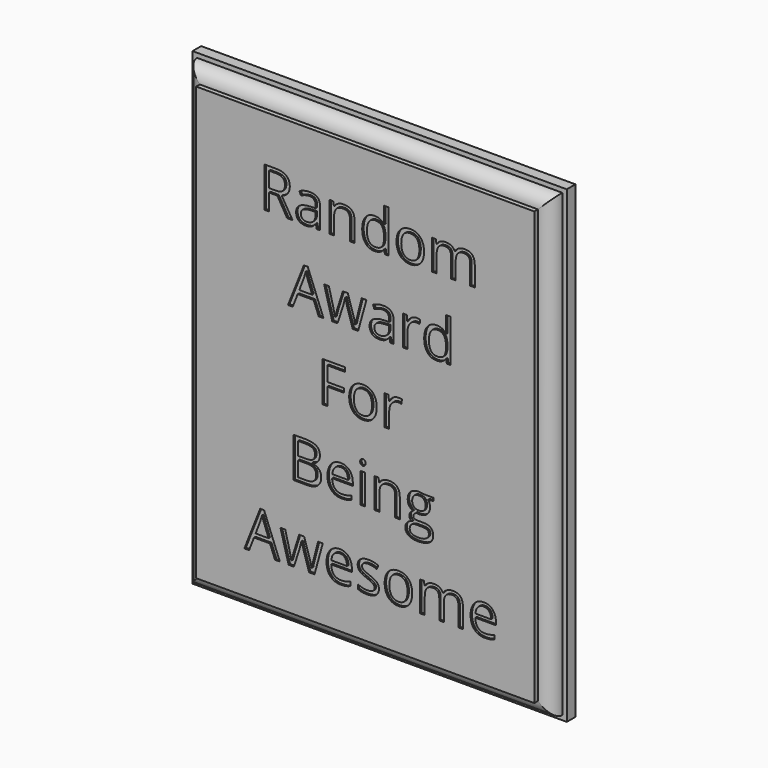
from build123d import *

# Parameters (mm, degrees)
F0_W         = 263.525
F0_H         = 330.2
F1_DEPTH     = 20.32
F4_TEXT_SIZE = 39.4429080188
F5_DEPTH     = 1.27


# Not quite as in the source:
# - Text() gives the source's letters only with a copy of the font that has no kerning and outlines rounded to 1/6400 em; it was checked with that copy


with BuildPart() as f1:
    # F0 (on Front) → F1 (new body)
    with BuildSketch(Plane.XZ):
        Rectangle(F0_W, F0_H)
    extrude(amount=-F1_DEPTH)

    # F3: sweep along a path in F3_path
    with BuildLine(Plane(origin=(131.7625, 0, 165.1), x_dir=(0, 0, -1), z_dir=(0, 1, 0))) as f3_path:
        Line((0, 0), (0, 263.525))
        Line((0, 263.525), (330.2, 263.525))
        Line((330.2, 263.525), (330.2, 0))
        Line((330.2, 0), (0, 0))
    # F2 (on face) → F3 (sweep, cut)
    with BuildSketch(Plane.YZ.offset(131.7625)):
        with BuildLine():
            Line((12.7, 161.925), (12.7, 165.1))
            Line((12.7, 165.1), (0, 165.1))
            Line((0, 165.1), (0, 152.4))
            Line((0, 152.4), (3.175, 152.4))
            ThreePointArc((3.175, 152.4), (5.9648079092, 159.1351920908), (12.7, 161.925))
        make_face()
    sweep(path=f3_path.line, transition=Transition.RIGHT, mode=Mode.SUBTRACT)

    # F4 (on face) → F5 (cut)
    with BuildSketch(Plane.XZ):
        with Locations((-74.8742776195, 91.6271954775)):
            Text('Random', F4_TEXT_SIZE, font='Open Sans', text_align=(TextAlign.LEFT, TextAlign.BOTTOM))
        with Locations((-54.3762913585, 37.9848405719)):
            Text('Award', F4_TEXT_SIZE, font='Open Sans', text_align=(TextAlign.LEFT, TextAlign.BOTTOM))
        with Locations((-33.8783050975, -15.6575143337)):
            Text('For', F4_TEXT_SIZE, font='Open Sans', text_align=(TextAlign.LEFT, TextAlign.BOTTOM))
        with Locations((-54.3762913585, -69.2998692393)):
            Text('Being', F4_TEXT_SIZE, font='Open Sans', text_align=(TextAlign.LEFT, TextAlign.BOTTOM))
        with Locations((-85.12327075, -122.9422241449)):
            Text('Awesome', F4_TEXT_SIZE, font='Open Sans', text_align=(TextAlign.LEFT, TextAlign.BOTTOM))
    extrude(amount=-F5_DEPTH, mode=Mode.SUBTRACT)


solid = f1.part
